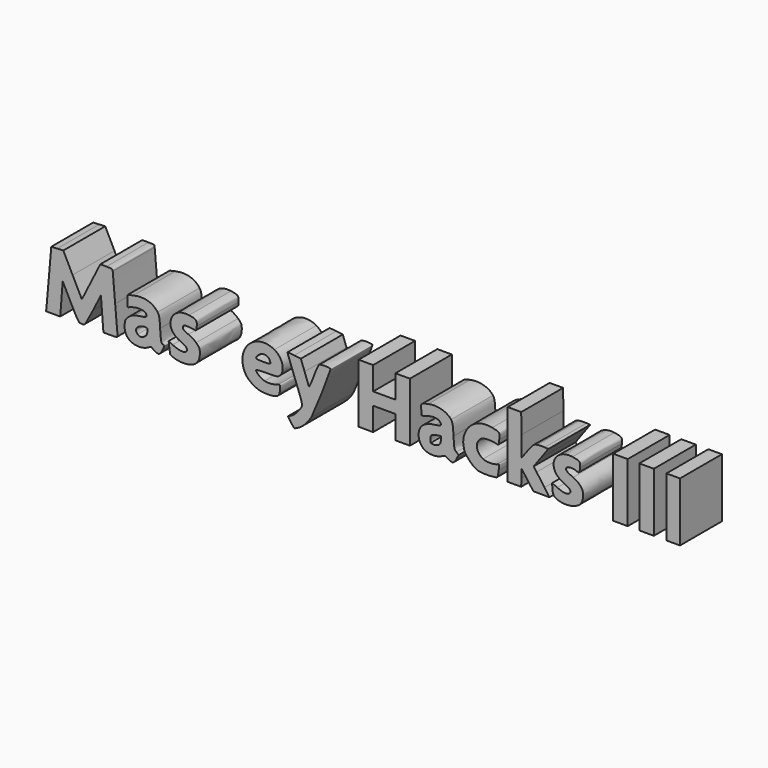
from build123d import *

# Parameters (mm, degrees)
F1_DEPTH = 6.35


# Not quite as in the source:
# - ends of sketch curves that miss each other by under 0.0002 mm in the source are joined


with BuildPart() as f1:
    # F0 (on Front) → F1 (new body)
    with BuildSketch(Plane.XZ):
        with BuildLine():
            add(Edge.make_bspline(
                [(-8.6592236118, -4.0772044411), (-8.1932667757, -3.836638873), (-7.5012651934, -3.0274957769), (-7.3931785155, -2.5968478734)],
                knots=[0, 0, 0, 0, 1, 1, 1, 1], degree=3))
            Line((-8.6592236118, -4.0772044411), (-9.0974985545, -4.3034791364))
            Line((-9.0974985545, -4.3034791364), (-8.7415782715, -4.8207932469))
            add(Edge.make_bspline(
                [(-8.3279583402, -5.3381061842), (-8.3596925015, -5.3381061842), (-8.5458211187, -5.1053154797), (-8.7415782715, -4.8207932469)],
                knots=[0, 0, 0, 0, 1, 1, 1, 1], degree=3))
            add(Edge.make_bspline(
                [(-7.8349801278, -5.1134047637), (-8.0743842179, -5.236990721), (-8.2962241788, -5.3381061842), (-8.3279583402, -5.3381061842)],
                knots=[0, 0, 0, 0, 1, 1, 1, 1], degree=3))
            add(Edge.make_bspline(
                [(-6.2486169838, -3.4609699436), (-6.6466637236, -4.1583389623), (-7.2968591353, -4.835615584), (-7.8349801278, -5.1134047637)],
                knots=[0, 0, 0, 0, 1, 1, 1, 1], degree=3))
            add(Edge.make_bspline(
                [(-3.9387304471, 2.3869382865), (-3.9387304471, 2.1449953697), (-5.9383169775, -2.9173289973), (-6.2486169838, -3.4609699436)],
                knots=[0, 0, 0, 0, 1, 1, 1, 1], degree=3))
            add(Edge.make_bspline(
                [(-5.3298479579, 2.4179063416), (-5.0860126531, 2.5724063863), (-3.9387304471, 2.5468667746), (-3.9387304471, 2.3869382865)],
                knots=[0, 0, 0, 0, 1, 1, 1, 1], degree=3))
            add(Edge.make_bspline(
                [(-5.9958101409, 0.9238595846), (-5.7171164161, 1.690089), (-5.4174327885, 2.3624099819), (-5.3298479579, 2.4179063416)],
                knots=[0, 0, 0, 0, 1, 1, 1, 1], degree=3))
            add(Edge.make_bspline(
                [(-6.5654623294, -0.2933025376), (-6.5308467639, -0.390092375), (-6.2745038657, 0.1576301694), (-5.9958101409, 0.9238595846)],
                knots=[0, 0, 0, 0, 1, 1, 1, 1], degree=3))
            add(Edge.make_bspline(
                [(-7.0836328833, 1.1145496429), (-6.8332534123, 0.437020781), (-6.6000767217, -0.1965127002), (-6.5654623294, -0.2933025376)],
                knots=[0, 0, 0, 0, 1, 1, 1, 1], degree=3))
            Line((-7.0836328833, 1.1145496429), (-7.5388689251, 2.3464203007))
            Line((-7.5388689251, 2.3464203007), (-8.3250476058, 2.4487781935))
            add(Edge.make_bspline(
                [(-9.1636593945, 2.4987041515), (-9.134821889, 2.527541657), (-8.757447112, 2.5050746826), (-8.3250476058, 2.4487781935)],
                knots=[0, 0, 0, 0, 1, 1, 1, 1], degree=3))
            add(Edge.make_bspline(
                [(-8.2721252691, 0.0542457177), (-8.7913071302, 1.3698601161), (-9.1924980732, 2.469866646), (-9.1636593945, 2.4987041515)],
                knots=[0, 0, 0, 0, 1, 1, 1, 1], degree=3))
            add(Edge.make_bspline(
                [(-7.3931785155, -2.5968478734), (-7.3513547468, -2.4302086233), (-7.6649362219, -1.4843795053), (-8.2721252691, 0.0542457177)],
                knots=[0, 0, 0, 0, 1, 1, 1, 1], degree=3))
        make_face()
    extrude(amount=F1_DEPTH)


with BuildPart() as f1b:
    # F0 (on Front) → F1, piece 2 (new body)
    with BuildSketch(Plane.XZ):
        with BuildLine():
            add(Edge.make_bspline(
                [(-28.1086897526, -2.541783255), (-28.6768144215, -2.2426217059), (-28.9540838692, -1.6753229769), (-28.8906624749, -0.9418519355)],
                knots=[0, 0, 0, 0, 1, 1, 1, 1], degree=3))
            add(Edge.make_bspline(
                [(-26.0923251438, -2.4970217681), (-26.6709441775, -2.8222238897), (-27.5395009821, -2.8415044253), (-28.1086897526, -2.541783255)],
                knots=[0, 0, 0, 0, 1, 1, 1, 1], degree=3))
            add(Edge.make_bspline(
                [(-25.54840732, -2.3621377971), (-25.6021685019, -2.2793560889), (-25.7862768512, -2.3250127351), (-26.0923251438, -2.4970217681)],
                knots=[0, 0, 0, 0, 1, 1, 1, 1], degree=3))
            add(Edge.make_bspline(
                [(-24.7729001588, -2.7570438534), (-24.9958933853, -2.7570438534), (-25.4382194226, -2.5318004098), (-25.54840732, -2.3621377971)],
                knots=[0, 0, 0, 0, 1, 1, 1, 1], degree=3))
            add(Edge.make_bspline(
                [(-24.2939265561, -2.1704387782), (-24.457856864, -2.4939397451), (-24.672685721, -2.7570438534), (-24.7729001588, -2.7570438534)],
                knots=[0, 0, 0, 0, 1, 1, 1, 1], degree=3))
            add(Edge.make_bspline(
                [(-24.1677055688, -1.583833703), (-24.0347034269, -1.583833703), (-24.0627713066, -1.7142759004), (-24.2939265561, -2.1704387782)],
                knots=[0, 0, 0, 0, 1, 1, 1, 1], degree=3))
            add(Edge.make_bspline(
                [(-24.5941956155, 0.0300576441), (-24.5264579811, -1.3330037193), (-24.4601727808, -1.583833703), (-24.1677055688, -1.583833703)],
                knots=[0, 0, 0, 0, 1, 1, 1, 1], degree=3))
            add(Edge.make_bspline(
                [(-24.8982858205, 1.6725518546), (-24.703915402, 1.4101680973), (-24.6476881323, 1.1064673981), (-24.5941956155, 0.0300576441)],
                knots=[0, 0, 0, 0, 1, 1, 1, 1], degree=3))
            add(Edge.make_bspline(
                [(-27.8135570072, 2.4992062854), (-26.542722867, 2.7830726938), (-25.5024210017, 2.4880842532), (-24.8982858205, 1.6725518546)],
                knots=[0, 0, 0, 0, 1, 1, 1, 1], degree=3))
            Line((-27.8135570072, 2.4992062854), (-28.5174830974, 2.3419703146))
            Line((-28.5174830974, 2.3419703146), (-28.5531146629, 1.6546287231))
            add(Edge.make_bspline(
                [(-28.3771331403, 1.0583235464), (-28.569399993, 0.9756110576), (-28.5854882238, 1.0301301333), (-28.5531146629, 1.6546287231)],
                knots=[0, 0, 0, 0, 1, 1, 1, 1], degree=3))
            add(Edge.make_bspline(
                [(-26.2523920707, 0.91676049), (-26.3204734557, 1.3870464716), (-27.439670184, 1.4616145356), (-28.3771331403, 1.0583235464)],
                knots=[0, 0, 0, 0, 1, 1, 1, 1], degree=3))
            add(Edge.make_bspline(
                [(-26.7216761309, 0.5902913015), (-26.2928525692, 0.6563618043), (-26.2218475444, 0.7057586445), (-26.2523920707, 0.91676049)],
                knots=[0, 0, 0, 0, 1, 1, 1, 1], degree=3))
            add(Edge.make_bspline(
                [(-27.6025715866, 0.4495401065), (-27.3959810112, 0.4841369007), (-26.9995779388, 0.5474738238), (-26.7216761309, 0.5902913015)],
                knots=[0, 0, 0, 0, 1, 1, 1, 1], degree=3))
            add(Edge.make_bspline(
                [(-28.4092075326, 0.0140550576), (-28.1721486896, 0.2189761549), (-27.809162162, 0.4149444856), (-27.6025715866, 0.4495401065)],
                knots=[0, 0, 0, 0, 1, 1, 1, 1], degree=3))
            add(Edge.make_bspline(
                [(-28.8906624749, -0.9418519355), (-28.8477863367, -0.4459887994), (-28.7755998894, -0.302667101), (-28.4092075326, 0.0140550576)],
                knots=[0, 0, 0, 0, 1, 1, 1, 1], degree=3))
        make_face()
        with BuildLine():
            add(Edge.make_bspline(
                [(-26.2213454105, -1.1511749173), (-26.0307668072, -0.6499138413), (-26.0846805065, -0.4106235526), (-26.3881981849, -0.4106235526)],
                knots=[0, 0, 0, 0, 1, 1, 1, 1], degree=3))
            add(Edge.make_bspline(
                [(-26.686813018, -1.5620026085), (-26.4871842717, -1.4924124752), (-26.2823464723, -1.3116184447), (-26.2213454105, -1.1511749173)],
                knots=[0, 0, 0, 0, 1, 1, 1, 1], degree=3))
            add(Edge.make_bspline(
                [(-27.2994821299, -1.4788736301), (-27.0897309264, -1.6487192636), (-26.9787604979, -1.6637762426), (-26.686813018, -1.5620026085)],
                knots=[0, 0, 0, 0, 1, 1, 1, 1], degree=3))
            add(Edge.make_bspline(
                [(-26.3881981849, -0.4106235526), (-27.2836742963, -0.4106235526), (-27.8291090809, -1.0500078329), (-27.2994821299, -1.4788736301)],
                knots=[0, 0, 0, 0, 1, 1, 1, 1], degree=3))
        make_face(mode=Mode.SUBTRACT)
    extrude(amount=F1_DEPTH)


with BuildPart() as f1c:
    # F0 (on Front) → F1, piece 3 (new body)
    with BuildSketch(Plane.XZ):
        with BuildLine():
            add(Edge.make_bspline(
                [(-22.8654739786, -2.5867371483), (-23.112249348, -2.4987323085), (-23.3315317108, -2.4086590992), (-23.3527668145, -2.3865745914)],
                knots=[0, 0, 0, 0, 1, 1, 1, 1], degree=3))
            add(Edge.make_bspline(
                [(-20.5960584993, -2.5212509041), (-21.1415988728, -2.7995645089), (-22.1843046456, -2.8296526564), (-22.8654739786, -2.5867371483)],
                knots=[0, 0, 0, 0, 1, 1, 1, 1], degree=3))
            add(Edge.make_bspline(
                [(-19.7770674771, -1.043549311), (-19.7770674771, -1.7734279829), (-20.0320682229, -2.2335246344), (-20.5960584993, -2.5212509041)],
                knots=[0, 0, 0, 0, 1, 1, 1, 1], degree=3))
            add(Edge.make_bspline(
                [(-20.2236886368, -0.0667521379), (-19.8299041695, -0.4413510997), (-19.7770674771, -0.5569087799), (-19.7770674771, -1.043549311)],
                knots=[0, 0, 0, 0, 1, 1, 1, 1], degree=3))
            add(Edge.make_bspline(
                [(-21.163936794, 0.5210191082), (-20.8924418867, 0.4314187025), (-20.4693306852, 0.1669208206), (-20.2236886368, -0.0667521379)],
                knots=[0, 0, 0, 0, 1, 1, 1, 1], degree=3))
            add(Edge.make_bspline(
                [(-21.814641379, 1.171410446), (-21.9223573225, 0.8907081854), (-21.7440305529, 0.7124682333), (-21.163936794, 0.5210191082)],
                knots=[0, 0, 0, 0, 1, 1, 1, 1], degree=3))
            add(Edge.make_bspline(
                [(-21.138021755, 1.3198496871), (-21.6302690574, 1.365493428), (-21.750267338, 1.3391677654), (-21.814641379, 1.171410446)],
                knots=[0, 0, 0, 0, 1, 1, 1, 1], degree=3))
            add(Edge.make_bspline(
                [(-20.3636725523, 1.2187870183), (-20.4604623897, 1.2438549996), (-20.8089198829, 1.2893321446), (-21.138021755, 1.3198496871)],
                knots=[0, 0, 0, 0, 1, 1, 1, 1], degree=3))
            add(Edge.make_bspline(
                [(-20.1522354458, 1.7230784961), (-20.1793354271, 1.3027970775), (-20.2291640086, 1.1839508893), (-20.3636725523, 1.2187870183)],
                knots=[0, 0, 0, 0, 1, 1, 1, 1], degree=3))
            add(Edge.make_bspline(
                [(-21.0759401667, 2.5796568251), (-20.2135755653, 2.4503502951), (-20.1114464485, 2.3556429057), (-20.1522354458, 1.7230784961)],
                knots=[0, 0, 0, 0, 1, 1, 1, 1], degree=3))
            add(Edge.make_bspline(
                [(-23.2783723857, 1.4199972519), (-23.0475479815, 2.2559775303), (-22.132058078, 2.7380155579), (-21.0759401667, 2.5796568251)],
                knots=[0, 0, 0, 0, 1, 1, 1, 1], degree=3))
            add(Edge.make_bspline(
                [(-22.0317462637, -0.6026287794), (-23.0822245539, -0.1319837955), (-23.5136303511, 0.5679639391), (-23.2783723857, 1.4199972519)],
                knots=[0, 0, 0, 0, 1, 1, 1, 1], degree=3))
            add(Edge.make_bspline(
                [(-21.4312175305, -1.4218966792), (-21.1906449231, -1.132024608), (-21.3571539469, -0.9048664855), (-22.0317462637, -0.6026287794)],
                knots=[0, 0, 0, 0, 1, 1, 1, 1], degree=3))
            add(Edge.make_bspline(
                [(-23.0771879627, -1.2241509351), (-22.3981386205, -1.5705764283), (-21.6310903046, -1.662728566), (-21.4312175305, -1.4218966792)],
                knots=[0, 0, 0, 0, 1, 1, 1, 1], degree=3))
            Line((-23.0771879627, -1.2241509351), (-23.5608532329, -0.9774037227))
            Line((-23.5608532329, -0.9774037227), (-23.4761146101, -1.6619120117))
            add(Edge.make_bspline(
                [(-23.3527668145, -2.3865745914), (-23.3740007451, -2.3644900835), (-23.4295076637, -2.0383916293), (-23.4761146101, -1.6619120117)],
                knots=[0, 0, 0, 0, 1, 1, 1, 1], degree=3))
        make_face()
    extrude(amount=F1_DEPTH)


with BuildPart() as f1d:
    # F0 (on Front) → F1, piece 4 (new body)
    with BuildSketch(Plane.XZ):
        with BuildLine():
            add(Edge.make_bspline(
                [(-13.0311091125, -2.477431505), (-14.0878981, -1.977834041), (-14.6170510741, -1.1598601921), (-14.612366446, -0.0330962583)],
                knots=[0, 0, 0, 0, 1, 1, 1, 1], degree=3))
            add(Edge.make_bspline(
                [(-11.6700938277, -2.7558964538), (-12.2387945427, -2.7550752067), (-12.6003262898, -2.6810843622), (-13.0311091125, -2.477431505)],
                knots=[0, 0, 0, 0, 1, 1, 1, 1], degree=3))
            add(Edge.make_bspline(
                [(-10.1113809004, -2.1489303165), (-10.2018342298, -2.6012004831), (-10.6031530527, -2.7574744215), (-11.6700938277, -2.7558964538)],
                knots=[0, 0, 0, 0, 1, 1, 1, 1], degree=3))
            add(Edge.make_bspline(
                [(-10.2353575366, -1.2819514796), (-10.0190539544, -1.1989480347), (-9.9783341765, -1.4837002167), (-10.1113809004, -2.1489303165)],
                knots=[0, 0, 0, 0, 1, 1, 1, 1], degree=3))
            add(Edge.make_bspline(
                [(-11.9377675895, -1.4608003277), (-11.4913716862, -1.5810015737), (-10.8349641267, -1.5120426275), (-10.2353575366, -1.2819514796)],
                knots=[0, 0, 0, 0, 1, 1, 1, 1], degree=3))
            add(Edge.make_bspline(
                [(-12.972448605, -0.6281320217), (-12.972448605, -0.8627130448), (-12.3758383936, -1.3428399132), (-11.9377675895, -1.4608003277)],
                knots=[0, 0, 0, 0, 1, 1, 1, 1], degree=3))
            add(Edge.make_bspline(
                [(-11.6437071582, -0.5279422212), (-12.3745150126, -0.5279422212), (-12.972448605, -0.5730275141), (-12.972448605, -0.6281320217)],
                knots=[0, 0, 0, 0, 1, 1, 1, 1], degree=3))
            add(Edge.make_bspline(
                [(-10.0305432014, -0.2251883027), (-10.303826081, -0.516083413), (-10.3670140065, -0.5279422212), (-11.6437071582, -0.5279422212)],
                knots=[0, 0, 0, 0, 1, 1, 1, 1], degree=3))
            add(Edge.make_bspline(
                [(-10.7413337442, 2.2690025093), (-9.7895541044, 1.7422147269), (-9.4154678355, 0.4295310074), (-10.0305432014, -0.2251883027)],
                knots=[0, 0, 0, 0, 1, 1, 1, 1], degree=3))
            add(Edge.make_bspline(
                [(-14.612366446, -0.0330962583), (-14.6040014576, 1.9801910202), (-12.4904657181, 3.237105022), (-10.7413337442, 2.2690025093)],
                knots=[0, 0, 0, 0, 1, 1, 1, 1], degree=3))
        make_face()
        with BuildLine():
            add(Edge.make_bspline(
                [(-11.2126333794, 0.6778233376), (-11.2126333794, 0.7602554292), (-11.2948190969, 0.9450360279), (-11.3952670035, 1.0884468902)],
                knots=[0, 0, 0, 0, 1, 1, 1, 1], degree=3))
            add(Edge.make_bspline(
                [(-12.0925409922, 0.5279469141), (-11.4567291369, 0.5279469141), (-11.2126333794, 0.5695243086), (-11.2126333794, 0.6778233376)],
                knots=[0, 0, 0, 0, 1, 1, 1, 1], degree=3))
            add(Edge.make_bspline(
                [(-12.6844783075, 1.0612237219), (-13.1395794301, 0.6061237725), (-13.0528041146, 0.5279469141), (-12.0925409922, 0.5279469141)],
                knots=[0, 0, 0, 0, 1, 1, 1, 1], degree=3))
            add(Edge.make_bspline(
                [(-11.3952670035, 1.0884468902), (-11.6533814491, 1.4569557181), (-12.3024529255, 1.4432502771), (-12.6844783075, 1.0612237219)],
                knots=[0, 0, 0, 0, 1, 1, 1, 1], degree=3))
        make_face(mode=Mode.SUBTRACT)
    extrude(amount=F1_DEPTH)


with BuildPart() as f1e:
    # F0 (on Front) → F1, piece 5 (new body)
    with BuildSketch(Plane.XZ):
        with BuildLine():
            add(Edge.make_bspline(
                [(7.5903693311, -2.5831037165), (7.0863957932, -2.3640114137), (6.7384709375, -1.7720130915), (6.7379207019, -1.1326487558)],
                knots=[0, 0, 0, 0, 1, 1, 1, 1], degree=3))
            add(Edge.make_bspline(
                [(9.4794899134, -2.5300969087), (8.9580695674, -2.7959322502), (8.1331409287, -2.8190914186), (7.5903693311, -2.5831037165)],
                knots=[0, 0, 0, 0, 1, 1, 1, 1], degree=3))
            add(Edge.make_bspline(
                [(10.2962131203, -2.5296276246), (9.9290757751, -2.3057650494), (9.9194331609, -2.3057697422), (9.4794899134, -2.5300969087)],
                knots=[0, 0, 0, 0, 1, 1, 1, 1], degree=3))
            add(Edge.make_bspline(
                [(11.3087439281, -2.2368917475), (10.992604855, -2.8156093309), (10.8383617433, -2.8602042219), (10.2962131203, -2.5296276246)],
                knots=[0, 0, 0, 0, 1, 1, 1, 1], degree=3))
            Line((11.3087439281, -2.2368917475), (11.3095968519, -1.4873453806))
            add(Edge.make_bspline(
                [(10.961911331, 0.0989356388), (11.021417723, -1.1549550004), (11.0478090854, -1.2753615582), (11.3095968519, -1.4873453806)],
                knots=[0, 0, 0, 0, 1, 1, 1, 1], degree=3))
            add(Edge.make_bspline(
                [(10.6586541053, 1.7757497658), (10.855253623, 1.5124274404), (10.908909216, 1.2157413647), (10.961911331, 0.0989356388)],
                knots=[0, 0, 0, 0, 1, 1, 1, 1], degree=3))
            add(Edge.make_bspline(
                [(7.9034967738, 2.5322063405), (9.0230630633, 2.766174948), (10.1502575651, 2.4566926692), (10.6586541053, 1.7757497658)],
                knots=[0, 0, 0, 0, 1, 1, 1, 1], degree=3))
            add(Edge.make_bspline(
                [(7.0579243293, 1.6286913931), (6.9906078773, 2.32090298), (7.0144885699, 2.3464203007), (7.9034967738, 2.5322063405)],
                knots=[0, 0, 0, 0, 1, 1, 1, 1], degree=3))
            Line((7.0579243293, 1.6286913931), (7.1163149985, 1.0282811541))
            Line((7.1163149985, 1.0282811541), (7.6494697924, 1.1887375867))
            add(Edge.make_bspline(
                [(9.2515035045, 1.1648322567), (9.0242045968, 1.3921311644), (8.35831046, 1.4020670812), (7.6494697924, 1.1887375867)],
                knots=[0, 0, 0, 0, 1, 1, 1, 1], degree=3))
            add(Edge.make_bspline(
                [(8.7612694307, 0.5839383685), (9.4714100151, 0.6662730837), (9.5989438245, 0.8173919367), (9.2515035045, 1.1648322567)],
                knots=[0, 0, 0, 0, 1, 1, 1, 1], degree=3))
            add(Edge.make_bspline(
                [(6.7379207019, -1.1326487558), (6.7370994548, -0.1367352966), (7.4005697394, 0.4261756264), (8.7612694307, 0.5839383685)],
                knots=[0, 0, 0, 0, 1, 1, 1, 1], degree=3))
        make_face()
        with BuildLine():
            add(Edge.make_bspline(
                [(9.2213156341, -1.3896662499), (9.3507078084, -1.2725681448), (9.4358652672, -1.0337870293), (9.4358652672, -0.7880663758)],
                knots=[0, 0, 0, 0, 1, 1, 1, 1], degree=3))
            add(Edge.make_bspline(
                [(8.2235485029, -1.5056169555), (8.3738813051, -1.6559509309), (9.0085762644, -1.582192382), (9.2213156341, -1.3896662499)],
                knots=[0, 0, 0, 0, 1, 1, 1, 1], degree=3))
            add(Edge.make_bspline(
                [(8.2978056661, -0.6647748943), (8.1386796538, -0.7968384681), (8.088050943, -1.3701193956), (8.2235485029, -1.5056169555)],
                knots=[0, 0, 0, 0, 1, 1, 1, 1], degree=3))
            add(Edge.make_bspline(
                [(8.9430712488, -0.4594326145), (8.6720350667, -0.5027733439), (8.3816655544, -0.5951765485), (8.2978056661, -0.6647748943)],
                knots=[0, 0, 0, 0, 1, 1, 1, 1], degree=3))
            Line((8.9430712488, -0.4594326145), (9.4358652672, -0.3806316083))
            Line((9.4358652672, -0.3806316083), (9.4358652672, -0.7880663758))
        make_face(mode=Mode.SUBTRACT)
        Polygon((11.3095968519, -1.4873453806), (11.3087439281, -2.2368917475), (11.5928883873, -1.7167408149), align=None)
    extrude(amount=F1_DEPTH)


with BuildPart() as f1f:
    # F0 (on Front) → F1, piece 6 (new body)
    with BuildSketch(Plane.XZ):
        with BuildLine():
            add(Edge.make_bspline(
                [(13.8940638386, -2.6098564275), (13.3222541166, -2.4189786557), (12.4175108182, -1.4847467201), (12.2619724825, -0.9245717232)],
                knots=[0, 0, 0, 0, 1, 1, 1, 1], degree=3))
            add(Edge.make_bspline(
                [(16.2515486843, -2.5582621648), (16.0769808799, -2.7328299691), (14.3740980233, -2.7700958163), (13.8940638386, -2.6098564275)],
                knots=[0, 0, 0, 0, 1, 1, 1, 1], degree=3))
            add(Edge.make_bspline(
                [(16.4416568302, -1.7568951055), (16.4029655327, -2.1317779841), (16.3174162217, -2.4923934541), (16.2515486843, -2.5582621648)],
                knots=[0, 0, 0, 0, 1, 1, 1, 1], degree=3))
            add(Edge.make_bspline(
                [(16.288253737, -1.1677828802), (16.4975884509, -1.0812480727), (16.5074715733, -1.1192061139), (16.4416568302, -1.7568951055)],
                knots=[0, 0, 0, 0, 1, 1, 1, 1], degree=3))
            add(Edge.make_bspline(
                [(14.5506731902, -1.1707276377), (14.9847632923, -1.3767163563), (15.7861127534, -1.3753601253), (16.288253737, -1.1677828802)],
                knots=[0, 0, 0, 0, 1, 1, 1, 1], degree=3))
            add(Edge.make_bspline(
                [(14.4757285258, 0.9951848957), (13.5362394356, 0.6060346085), (13.5818104374, -0.7109723904), (14.5506731902, -1.1707276377)],
                knots=[0, 0, 0, 0, 1, 1, 1, 1], degree=3))
            add(Edge.make_bspline(
                [(16.2527805549, 0.9478705036), (15.8632255102, 1.1133752595), (14.8276329104, 1.1409480444), (14.4757285258, 0.9951848957)],
                knots=[0, 0, 0, 0, 1, 1, 1, 1], degree=3))
            add(Edge.make_bspline(
                [(16.5109571806, 1.5451482715), (16.4528938371, 0.9825670206), (16.4091741608, 0.8814245735), (16.2527805549, 0.9478705036)],
                knots=[0, 0, 0, 0, 1, 1, 1, 1], degree=3))
            add(Edge.make_bspline(
                [(15.6639193966, 2.5316162158), (16.5775004871, 2.340687996), (16.5913948149, 2.3245070816), (16.5109571806, 1.5451482715)],
                knots=[0, 0, 0, 0, 1, 1, 1, 1], degree=3))
            add(Edge.make_bspline(
                [(12.4568814044, 1.1221191947), (13.0316276714, 2.2555446157), (14.3056459039, 2.8154779313), (15.6639193966, 2.5316162158)],
                knots=[0, 0, 0, 0, 1, 1, 1, 1], degree=3))
            add(Edge.make_bspline(
                [(12.2619724825, -0.9245717232), (12.0516217686, -0.1669876935), (12.1090656571, 0.4362089196), (12.4568814044, 1.1221191947)],
                knots=[0, 0, 0, 0, 1, 1, 1, 1], degree=3))
        make_face()
    extrude(amount=F1_DEPTH)


with BuildPart() as f1g:
    # F0 (on Front) → F1, piece 7 (new body)
    with BuildSketch(Plane.XZ):
        with BuildLine():
            add(Edge.make_bspline(
                [(23.4992925499, -2.5681452871), (23.0689015794, -2.3893985082), (22.933133008, -2.0794985666), (22.9290737008, -1.2665965051)],
                knots=[0, 0, 0, 0, 1, 1, 1, 1], degree=3))
            add(Edge.make_bspline(
                [(26.5104900913, -1.8846612105), (26.1881013277, -2.6562475033), (24.5866612599, -3.019742031), (23.4992925499, -2.5681452871)],
                knots=[0, 0, 0, 0, 1, 1, 1, 1], degree=3))
            add(Edge.make_bspline(
                [(25.4550045403, 0.4169659267), (26.5863498596, -0.0960096527), (26.9377063551, -0.8621897931), (26.5104900913, -1.8846612105)],
                knots=[0, 0, 0, 0, 1, 1, 1, 1], degree=3))
            add(Edge.make_bspline(
                [(24.6411087698, 1.1626254484), (24.5335512096, 0.8823349846), (24.6363338045, 0.7881684451), (25.4550045403, 0.4169659267)],
                knots=[0, 0, 0, 0, 1, 1, 1, 1], degree=3))
            add(Edge.make_bspline(
                [(25.8785697741, 1.2223676557), (25.5085756622, 1.4203820649), (24.7255130277, 1.3825777142), (24.6411087698, 1.1626254484)],
                knots=[0, 0, 0, 0, 1, 1, 1, 1], degree=3))
            add(Edge.make_bspline(
                [(26.2991409756, 1.7424282511), (26.2282051702, 1.113081957), (26.1842743162, 1.0587588074), (25.8785697741, 1.2223676557)],
                knots=[0, 0, 0, 0, 1, 1, 1, 1], degree=3))
            add(Edge.make_bspline(
                [(25.3831829613, 2.5796591715), (26.2559070083, 2.4487981381), (26.3672845407, 2.3469940005), (26.2991409756, 1.7424282511)],
                knots=[0, 0, 0, 0, 1, 1, 1, 1], degree=3))
            add(Edge.make_bspline(
                [(23.5515332514, -0.0451721104), (22.4046053548, 1.2076884503), (23.553445584, 2.854019058), (25.3831829613, 2.5796591715)],
                knots=[0, 0, 0, 0, 1, 1, 1, 1], degree=3))
            add(Edge.make_bspline(
                [(24.4273768642, -0.602626433), (24.0865499299, -0.4499260927), (23.6924205388, -0.1990714715), (23.5515332514, -0.0451721104)],
                knots=[0, 0, 0, 0, 1, 1, 1, 1], degree=3))
            add(Edge.make_bspline(
                [(25.0383213572, -1.4093445038), (25.2684265836, -1.1320844418), (25.0934610611, -0.9010512061), (24.4273768642, -0.602626433)],
                knots=[0, 0, 0, 0, 1, 1, 1, 1], degree=3))
            add(Edge.make_bspline(
                [(23.5437184986, -1.2947805326), (24.2436943903, -1.6206654625), (24.8259022738, -1.6652932034), (25.0383213572, -1.4093445038)],
                knots=[0, 0, 0, 0, 1, 1, 1, 1], degree=3))
            Line((23.5437184986, -1.2947805326), (22.9277831697, -1.008020988))
            Line((22.9277831697, -1.008020988), (22.9290737008, -1.2665965051))
        make_face()
    extrude(amount=F1_DEPTH)


with BuildPart() as f1h:
    # F0 (on Front) → F1, piece 8 (new body)
    with BuildSketch(Plane.XZ):
        with BuildLine():
            add(Edge.make_bspline(
                [(-38.3519185028, -2.0237875094), (-38.3176877502, -1.6850230785), (-38.1763175403, -0.0879907613), (-38.0377624481, 1.5251731955)],
                knots=[0, 0, 0, 0, 1, 1, 1, 1], degree=3))
            Line((-38.3519185028, -2.0237875094), (-38.4141559814, -2.6397228383))
            Line((-38.4141559814, -2.6397228383), (-37.5571831605, -2.6397228383))
            Line((-37.5571831605, -2.6397228383), (-36.700210193, -2.6397228383))
            Line((-36.700210193, -2.6397228383), (-36.5507276748, -0.7073565567))
            Line((-36.5507276748, -0.7073565567), (-36.4012451566, 1.2250097249))
            Line((-36.4012451566, 1.2250097249), (-35.4369649627, -0.6780263029))
            add(Edge.make_bspline(
                [(-34.0761466305, -2.5810623308), (-34.4707211082, -2.5810623308), (-34.4774600274, -2.5716414533), (-35.4369649627, -0.6780263029)],
                knots=[0, 0, 0, 0, 1, 1, 1, 1], degree=3))
            add(Edge.make_bspline(
                [(-32.7254632209, -0.6809933514), (-33.6756772117, -2.5732334995), (-33.6812423341, -2.5810623308), (-34.0761466305, -2.5810623308)],
                knots=[0, 0, 0, 0, 1, 1, 1, 1], degree=3))
            Line((-32.7254632209, -0.6809933514), (-31.7713185361, 1.2190768012))
            Line((-31.7713185361, 1.2190768012), (-31.6189525606, -0.7103236052))
            Line((-31.6189525606, -0.7103236052), (-31.4665877584, -2.6397228383))
            Line((-31.4665877584, -2.6397228383), (-30.6079715634, -2.6397228383))
            add(Edge.make_bspline(
                [(-29.7506970809, -2.434411062), (-29.7495238708, -2.611366349), (-29.8679430105, -2.6397228383), (-30.6079715634, -2.6397228383)],
                knots=[0, 0, 0, 0, 1, 1, 1, 1], degree=3))
            add(Edge.make_bspline(
                [(-30.0426562929, 0.8799076128), (-29.8828169688, -0.8300461814), (-29.7514350301, -2.3214895851), (-29.7506970809, -2.434411062)],
                knots=[0, 0, 0, 0, 1, 1, 1, 1], degree=3))
            add(Edge.make_bspline(
                [(-30.334617118, 4.2528867951), (-30.3339131919, 4.107702039), (-30.2024967902, 2.5898614069), (-30.0426562929, 0.8799076128)],
                knots=[0, 0, 0, 0, 1, 1, 1, 1], degree=3))
            add(Edge.make_bspline(
                [(-31.0894476235, 4.5168590789), (-30.3866642399, 4.5168590789), (-30.3358689333, 4.4990955041), (-30.334617118, 4.2528867951)],
                knots=[0, 0, 0, 0, 1, 1, 1, 1], degree=3))
            Line((-31.0894476235, 4.5168590789), (-31.8429359765, 4.5168590789))
            Line((-31.8429359765, 4.5168590789), (-32.9617349865, 2.279244634))
            Line((-32.9617349865, 2.279244634), (-34.0805337032, 0.041630189))
            Line((-34.0805337032, 0.041630189), (-35.203278219, 2.2847563752))
            Line((-35.203278219, 2.2847563752), (-36.3260227347, 4.5278813883))
            Line((-36.3260227347, 4.5278813883), (-37.0559333767, 4.4930405665))
            Line((-37.0559333767, 4.4930405665), (-37.7858440186, 4.4581985714))
            Line((-37.7858440186, 4.4581985714), (-38.0377624481, 1.5251731955))
        make_face()
    extrude(amount=F1_DEPTH)


with BuildPart() as f1i:
    # F0 (on Front) → F1, piece 9 (new body)
    with BuildSketch(Plane.XZ):
        Polygon((-0.536421011, 4.5168590789), (-0.536421011, 0.9385681203), (-0.536421011, -2.6397228383), (0.3434866018, -2.6397228383), (1.2233942146, -2.6397228383), (1.2233942146, -1.2318706579), (1.2233942146, 0.1759815226), (2.5725858875, 0.1759815226), (3.9217775604, 0.1759815226), (3.9217775604, -1.2318706579), (3.9217775604, -2.6397228383), (4.8016851732, -2.6397228383), (5.681592786, -2.6397228383), (5.681592786, 0.9385681203), (5.681592786, 4.5168590789), (4.8016851732, 4.5168590789), (3.9217775604, 4.5168590789), (3.9217775604, 3.1090068985), (3.9217775604, 1.701154718), (2.5725858875, 1.701154718), (1.2233942146, 1.701154718), (1.2233942146, 3.1090068985), (1.2233942146, 4.5168590789), (0.3434866018, 4.5168590789), align=None)
    extrude(amount=F1_DEPTH)


with BuildPart() as f1j:
    # F0 (on Front) → F1, piece 10 (new body)
    with BuildSketch(Plane.XZ):
        with BuildLine():
            add(Edge.make_bspline(
                [(19.9360749952, 1.4465516905), (20.5705587766, 2.305511636), (20.6862654545, 2.40643), (21.1092851456, 2.4698244104)],
                knots=[0, 0, 0, 0, 1, 1, 1, 1], degree=3))
            Line((19.9360749952, 1.4465516905), (19.2321700228, 0.4936105726))
            Line((19.2321700228, 0.4936105726), (19.2004593256, 2.9158577918))
            Line((19.2004593256, 2.9158577918), (19.1687486285, 5.3381061842))
            Line((19.1687486285, 5.3381061842), (18.3498819666, 5.3381061842))
            Line((18.3498819666, 5.3381061842), (17.5310153047, 5.3381061842))
            Line((17.5310153047, 5.3381061842), (17.5310153047, 1.3491916729))
            Line((17.5310153047, 1.3491916729), (17.5310153047, -2.6397134527))
            Line((17.5310153047, -2.6397134527), (18.3475179482, -2.6397134527))
            Line((18.3475179482, -2.6397134527), (19.1640205916, -2.6397134527))
            Line((19.1640205916, -2.6397134527), (19.1980953072, -1.6757183488))
            Line((19.1980953072, -1.6757183488), (19.2321700228, -0.7117220717))
            Line((19.2321700228, -0.7117220717), (19.936096113, -1.6718514481))
            Line((19.936096113, -1.6718514481), (20.6400222032, -2.6319796513))
            Line((20.6400222032, -2.6319796513), (21.6141303786, -2.6358512448))
            Line((21.6141303786, -2.6358512448), (22.5882397272, -2.6397228383))
            Line((22.5882397272, -2.6397228383), (21.9890942087, -1.7891454793))
            add(Edge.make_bspline(
                [(21.0334887306, -0.4539513767), (21.2295415324, -0.7204906443), (21.6595629417, -1.3213279319), (21.9890942087, -1.7891454793)],
                knots=[0, 0, 0, 0, 1, 1, 1, 1], degree=3))
            Line((21.0334887306, -0.4539513767), (20.677028771, 0.0306653669))
            Line((20.677028771, 0.0306653669), (21.5627074045, 1.2472033413))
            Line((21.5627074045, 1.2472033413), (22.448386038, 2.4637413158))
            Line((22.448386038, 2.4637413158), (22.0134887674, 2.5019480775))
            add(Edge.make_bspline(
                [(21.1092851456, 2.4698244104), (21.3674031108, 2.5085051491), (21.7742946819, 2.5229614445), (22.0134887674, 2.5019480775)],
                knots=[0, 0, 0, 0, 1, 1, 1, 1], degree=3))
        make_face()
    extrude(amount=F1_DEPTH)


with BuildPart() as f1k:
    # F0 (on Front) → F1, piece 11 (new body)
    with BuildSketch(Plane.XZ):
        Polygon((30.3190059438, 4.5168590789), (30.3190059438, 0.9385681203), (30.3190059438, -2.6397228383), (31.1989135566, -2.6397228383), (32.0788211694, -2.6397228383), (32.0788211694, 0.9385681203), (32.0788211694, 4.5168590789), (31.1989135566, 4.5168590789), align=None)
    extrude(amount=F1_DEPTH)


with BuildPart() as f1l:
    # F0 (on Front) → F1, piece 12 (new body)
    with BuildSketch(Plane.XZ):
        Polygon((33.4866733498, 4.5168590789), (33.4866733498, 0.9385681203), (33.4866733498, -2.6397228383), (34.3665809626, -2.6397228383), (35.2464885754, -2.6397228383), (35.2464885754, 0.9385681203), (35.2464885754, 4.5168590789), (34.3665809626, 4.5168590789), align=None)
    extrude(amount=F1_DEPTH)


with BuildPart() as f1m:
    # F0 (on Front) → F1, piece 13 (new body)
    with BuildSketch(Plane.XZ):
        Polygon((36.7716617709, 4.5168590789), (36.7716617709, 0.9385681203), (36.7716617709, -2.6397228383), (37.5929088761, -2.6397228383), (38.4141559814, -2.6397228383), (38.4141559814, 0.9385681203), (38.4141559814, 4.5168590789), (37.5929088761, 4.5168590789), align=None)
    extrude(amount=F1_DEPTH)


solid = Compound([f1.part, f1b.part, f1c.part, f1d.part, f1e.part, f1f.part, f1g.part, f1h.part, f1i.part, f1j.part, f1k.part, f1l.part, f1m.part])
